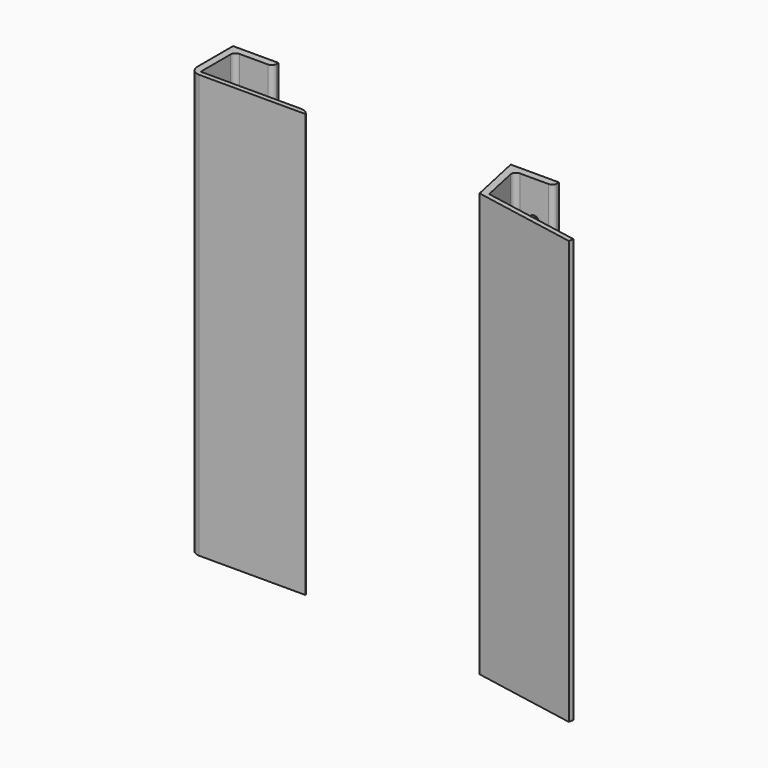
from build123d import *

# Parameters (mm, degrees)
F1_DEPTH    = 277.8125
F3_D        = 6.7564
F3_DEPTH    = 4.7635
F5_DEPTH    = 277.8125
F7_D        = 6.7564
F7_DEPTH    = 4.7635
F8_R        = 6.35
F9_T1_DEPTH = 305.3088065702


# Not quite as in the source:
# - a fillet or chamfer that OpenCascade refuses, or shapes differently, is made with other operations: its cross-section is extruded or revolved along the edge and cut away or added


with BuildPart() as f1:
    # F0 (on Top) → F1 (new body)
    with BuildSketch(Plane.XY):
        with BuildLine():
            Line((0, -1.5875), (0, 0))
            Line((0, 0), (-31.75, 0))
            Line((-31.75, 0), (-24.2357517976, -34.925))
            Line((-24.2357517976, -34.925), (44.45, -47.625))
            Line((44.45, -47.625), (45.0272727273, -44.5029203728))
            Line((45.0272727273, -44.5029203728), (-19.8859153776, -32.5004676464))
            Line((-19.8859153776, -32.5004676464), (-25.0270460191, -8.6053309912))
            ThreePointArc((-25.0270460191, -8.6053309912), (-24.392994354, -5.9424734835), (-21.9230765014, -4.7625))
            Line((-21.9230765014, -4.7625), (-3.175, -4.7625))
            ThreePointArc((-3.175, -4.7625), (-0.9299359697, -3.8325640303), (0, -1.5875))
        make_face()
    extrude(amount=F1_DEPTH)

    # F3 (through all, one way)
    with BuildSketch(Plane.XZ.offset(4.7625)):
        with Locations((-12.5490382507, 253.20625), (-12.5490382507, 24.60625)):
            Circle(F3_D / 2)
    extrude(amount=-F3_DEPTH, mode=Mode.SUBTRACT)


with BuildPart() as f5:
    # F4 (on Top) → F5 (new body)
    with BuildSketch(Plane.XY):
        with BuildLine():
            Line((-195.0523899696, 12.1864487154), (-195.0523899696, 13.7739487154))
            Line((-195.0523899696, 13.7739487154), (-224.925666471, 13.7739487154))
            Line((-224.925666471, 13.7739487154), (-224.925666471, -21.9502664761))
            Line((-224.925666471, -21.9502664761), (-148.725666471, -21.9502664761))
            Line((-148.725666471, -21.9502664761), (-148.725666471, -18.7752664761))
            Line((-148.725666471, -18.7752664761), (-220.150466471, -18.7752664761))
            Line((-220.150466471, -18.7752664761), (-220.150466471, 5.8364487154))
            ThreePointArc((-220.150466471, 5.8364487154), (-219.2205305013, 8.0815127456), (-216.975466471, 9.0114487154))
            Line((-216.975466471, 9.0114487154), (-198.2273899696, 9.0114487154))
            ThreePointArc((-198.2273899696, 9.0114487154), (-195.9823259393, 9.9413846851), (-195.0523899696, 12.1864487154))
        make_face()
    extrude(amount=F5_DEPTH)

    # F7 (through all, one way)
    with BuildSketch(Plane.XZ.offset(-9.0114487154)):
        with Locations((-207.6014282203, 253.20625), (-207.6014282203, 24.60625)):
            Circle(F7_D / 2)
    extrude(amount=-F7_DEPTH, mode=Mode.SUBTRACT)

    # F8
    f8_edges = [f5.edges().sort_by_distance(p)[0] for p in [
        (-224.925666, -21.950266, 138.90625),
    ]]
    fillet(f8_edges, radius=F8_R)

    # F9: fillet of radius 6.35 on 1 edges, made by hand

    # F9_s2 → F9_t1 (cut)
    with BuildSketch(Plane.XY.offset(-13.7481532851)):
        with BuildLine():
            ThreePointArc((-148.725666471, -21.9502664761), (-151.049927785, -19.6260051621), (-154.224927785, -18.7752664761))
            Line((-154.224927785, -18.7752664761), (-148.725666471, -18.7752664761))
            Line((-148.725666471, -18.7752664761), (-148.725666471, -21.9502664761))
        make_face()
    extrude(amount=F9_T1_DEPTH, mode=Mode.SUBTRACT)


solid = Compound([f1.part, f5.part])
